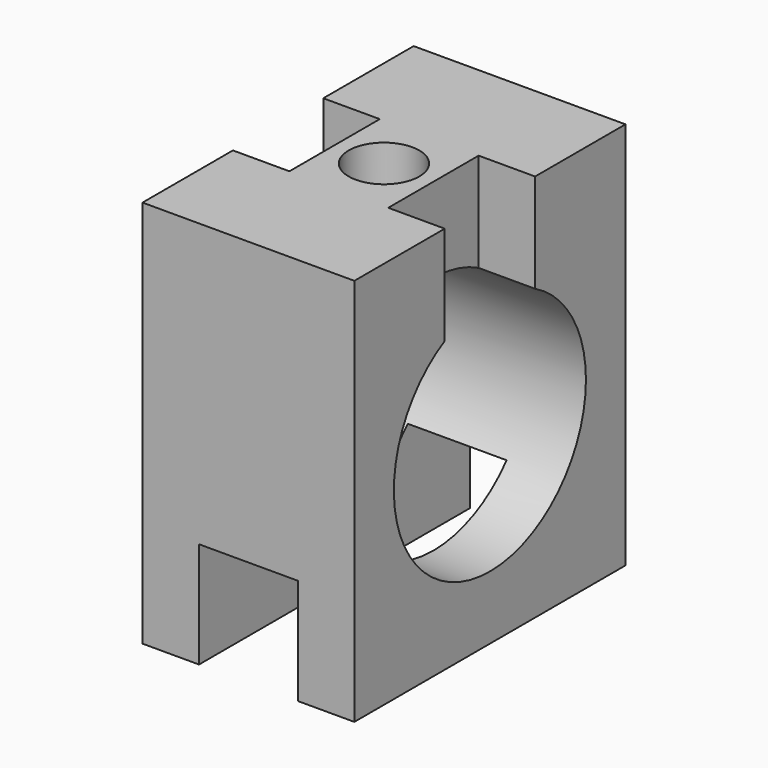
from build123d import *

# Parameters (mm, degrees)
F0_W     = 48
F0_H     = 55
F1_DEPTH = 15
F2_R     = 17
F3_DEPTH = 30.001
F4_W     = 8
F4_H     = 16
F5_REACH = 72.88954382
F6_R     = 5
F7_REACH = 69.1431356237
F8_W     = 14
F8_H     = 15
F9_DEPTH = 48.001


# Not quite as in the source:
# - a pattern or mirror of a feature is missing from the dataset's text; its kind, count and spacing are read off the source's solid


with BuildPart() as f1:
    # F0 (on Right) → F1 (new body, symmetric)
    with BuildSketch(Plane.YZ):
        Rectangle(F0_W, F0_H)
    extrude(amount=F1_DEPTH, both=True)

    # F2 (on face) → F3 (cut, through all)
    with BuildSketch(Plane.YZ.offset(15)):
        with Locations((0, -1.5)):
            Circle(F2_R)
    extrude(amount=-F3_DEPTH, mode=Mode.SUBTRACT)

    f5_end = f1.faces().sort_by_distance((0, -17, -1.5))[0]
    # F4 (on face) → F5 (cut, up to a face of the model that its end follows)
    with BuildSketch(Plane.XY.offset(27.5)):
        with Locations((11, 0)):
            Rectangle(F4_W, F4_H)
    f5_long = extrude(amount=-F5_REACH, mode=Mode.PRIVATE)
    f5 = split(f5_long, bisect_by=f5_end, keep=Keep.ALL, mode=Mode.PRIVATE).solids().sort_by_distance((11, 0, 27.5))[0]
    add(f5, mode=Mode.SUBTRACT)

    # F5_copies: F5 across plane
    add(f5.mirror(Plane(origin=(0, 0, 0), x_dir=(0, 0, -1), z_dir=(-1, 0, 0))), mode=Mode.SUBTRACT)

    f7_end = f1.faces().sort_by_distance((0, -17, -1.5))[0]
    # F6 (on face) → F7 (cut, up to a face of the model that its end follows)
    with BuildSketch(Plane.XY.offset(27.5)):
        Circle(F6_R)
    f7_long = extrude(amount=-F7_REACH, mode=Mode.PRIVATE)
    add(split(f7_long, bisect_by=f7_end, keep=Keep.ALL, mode=Mode.PRIVATE).solids().sort_by_distance((0, 0, 27.5))[0], mode=Mode.SUBTRACT)

    # F8 (on face) → F9 (cut, through all)
    with BuildSketch(Plane.XZ.offset(24)):
        with Locations((0, -20)):
            Rectangle(F8_W, F8_H)
    extrude(amount=-F9_DEPTH, mode=Mode.SUBTRACT)


solid = f1.part
